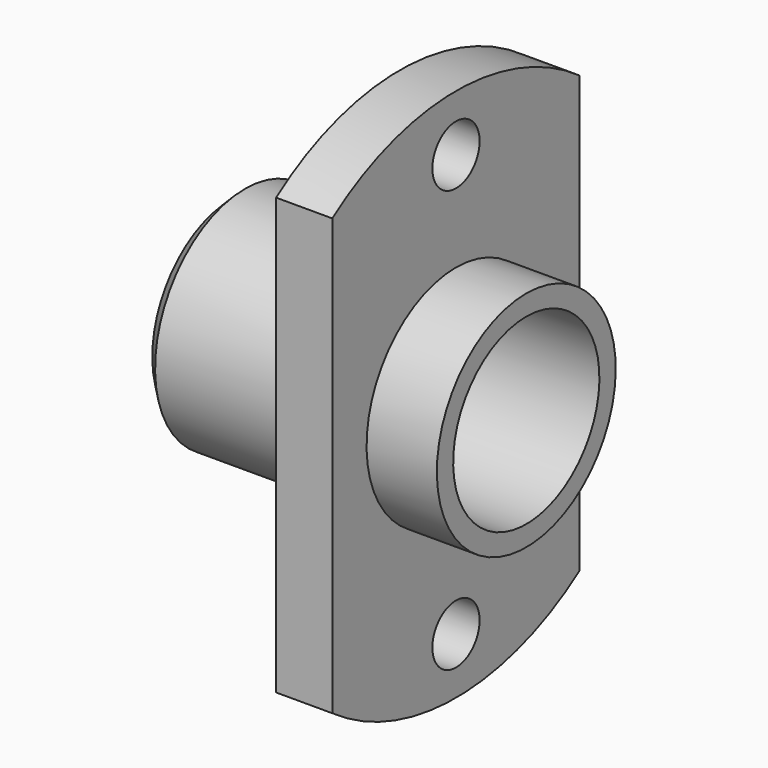
from build123d import *

# Parameters (mm, degrees)
F2_R     = 2.1
F3_DEPTH = 9.001
F4_SIZE  = 1


# Not quite as in the source:
# - a feature names something its author has since deleted; it is built from what else it names


with BuildPart() as f1:
    # F0 (on Front) → F1 (revolve)
    with BuildSketch(Plane.XZ):
        Polygon((0, 6.5), (20, 6.5), (20, 7.95), (15, 7.95), (15, 19), (11, 19), (11, 8), (-1, 8), (-1, 2.6), (0, 2.6), align=None)
    revolve(axis=Axis((12.5816260299, 0, 0), (1, 0, 0)))

    # F2 (on face) → F3 (cut, through all)
    with BuildSketch(Plane(origin=(11, 0, 0), x_dir=(0, -1, 0), z_dir=(-1, 0, 0))):
        with Locations((0, 15)):
            Circle(F2_R)
        with Locations((0, -15)):
            Circle(F2_R)
        with BuildLine():
            Line((-11, -15.4919333848), (-11, 15.4919333848))
            ThreePointArc((-11, 15.4919333848), (-19, 0), (-11, -15.4919333848))
        make_face()
        with BuildLine():
            ThreePointArc((19, 0), (16.8819430161, 8.7177978871), (11, 15.4919333848))
            Line((11, 15.4919333848), (11, -15.4919333848))
            ThreePointArc((11, -15.4919333848), (16.8819430161, -8.7177978871), (19, 0))
        make_face()
    extrude(amount=-F3_DEPTH, mode=Mode.SUBTRACT)

    # F4
    f4_edges = [f1.edges().sort_by_distance(p)[0] for p in [
        (-1, 0, -8),
    ]]
    chamfer(f4_edges, length=F4_SIZE)


solid = f1.part
